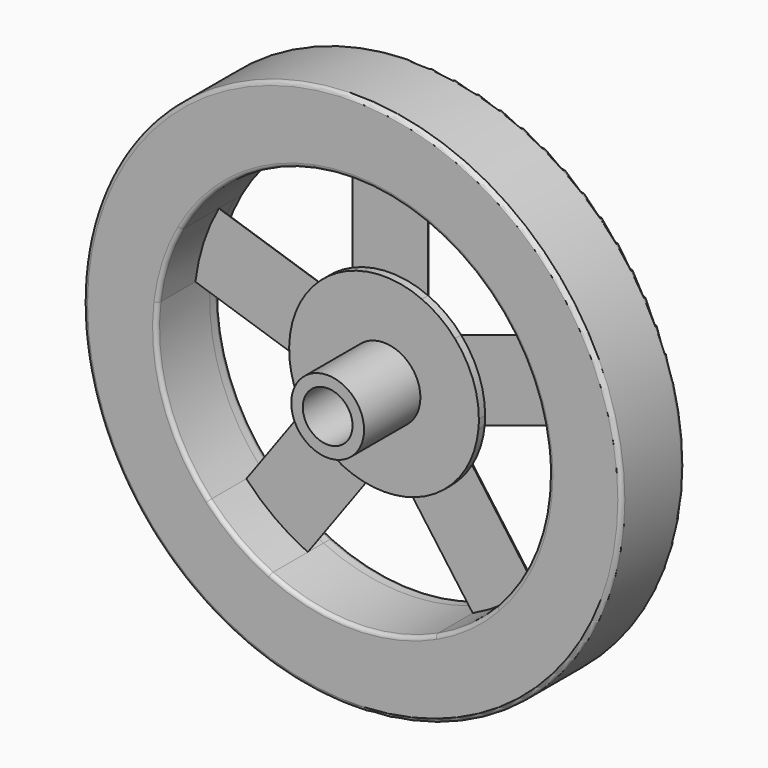
from build123d import *

# Parameters (mm, degrees)
F0_R          = 2.3622
F1_DEPTH      = 1.27
F2_T4_DEPTH   = 21.4195320699
F2_T9_DEPTH   = 21.4195320699
F2_T14_DEPTH  = 21.4195320699
F2_T19_DEPTH  = 21.4195320699
F2_T24_DEPTH  = 21.4195320699
F2_T29_DEPTH  = 21.4195320699
F2_T34_DEPTH  = 21.4195320699
F2_T39_DEPTH  = 21.4195320699
F2_T44_DEPTH  = 21.4195320699
F2_T49_DEPTH  = 21.4195320699
F2_T55_DEPTH  = 21.4195320699
F2_S57_R      = 2.3622
F2_T58_DEPTH  = 13
F2_T61_DEPTH  = 21.4195320699
F2_S63_R      = 2.3622
F2_T64_DEPTH  = 13
F2_T70_DEPTH  = 21.4195320699
F2_S72_R      = 2.3622
F2_T73_DEPTH  = 13
F2_T76_DEPTH  = 21.4195320699
F2_S78_R      = 2.3622
F2_T79_DEPTH  = 13
F2_T85_DEPTH  = 21.4195320699
F2_S87_R      = 2.3622
F2_T88_DEPTH  = 12
F2_T91_DEPTH  = 21.4195320699
F2_S93_R      = 2.3622
F2_T94_DEPTH  = 13
F2_T100_DEPTH = 21.4195320699
F2_S102_R     = 2.3622
F2_T103_DEPTH = 13
F2_T106_DEPTH = 21.4195320699
F2_S108_R     = 2.3622
F2_T109_DEPTH = 12
F2_T115_DEPTH = 21.4195320699
F2_S117_R     = 2.3622
F2_T118_DEPTH = 13
F2_T121_DEPTH = 21.4195320699
F2_S123_R     = 2.3622
F2_T124_DEPTH = 13
F0_R_2        = 17.4625
F3_DEPTH      = 4.318
F4_DEPTH      = 0.381
F5_DEPTH      = 0.762
F7_R          = 2.3622
F8_DEPTH      = 0.508
F7_R_2        = 1.6129
F9_DEPTH      = 5.08
F10_R         = 0.254


# Not quite as in the source:
# - a fillet or chamfer that OpenCascade refuses, or shapes differently, is made with other operations: its cross-section is extruded or revolved along the edge and cut away or added


with BuildPart() as f1:
    # F0 (on Front) → F1 (new body)
    with BuildSketch(Plane.XZ):
        with BuildLine():
            ThreePointArc((6.1303316445, -0.5987271324), (6.1522035895, -0.2997186064), (6.1595, 0))
            ThreePointArc((6.1595, 0), (5.7584751705, 2.1861847956), (4.607619503, 4.0876989573))
            Line((4.607619503, 4.0876989573), (2.4638, 3.3911297757))
            Line((2.4638, 3.3911297757), (2.4638, 5.6452749986))
            ThreePointArc((2.4638, 5.6452749986), (0, 6.1595), (-2.4638, 5.6452749986))
            Line((-2.4638, 5.6452749986), (-2.4638, 3.3911297757))
            Line((-2.4638, 3.3911297757), (-4.607619503, 4.0876989573))
            ThreePointArc((-4.607619503, 4.0876989573), (-5.8580326121, 1.9033901769), (-6.1303316445, -0.5987271324))
            Line((-6.1303316445, -0.5987271324), (-3.9865121415, -1.295296314))
            Line((-3.9865121415, -1.295296314), (-5.3114654601, -3.1189381072))
            ThreePointArc((-5.3114654601, -3.1189381072), (-3.6204632615, -4.9831401769), (-1.3249533186, -6.0153087164))
            Line((-1.3249533186, -6.0153087164), (0, -4.1916669232))
            Line((0, -4.1916669232), (1.3249533186, -6.0153087164))
            ThreePointArc((1.3249533186, -6.0153087164), (3.6204632615, -4.9831401769), (5.3114654601, -3.1189381072))
            Line((5.3114654601, -3.1189381072), (3.9865121415, -1.295296314))
            Line((3.9865121415, -1.295296314), (6.1303316445, -0.5987271324))
        make_face()
        Circle(F0_R, mode=Mode.SUBTRACT)
        with BuildLine():
            ThreePointArc((-2.4638, 5.6452749986), (0, 6.1595), (2.4638, 5.6452749986))
            Line((2.4638, 5.6452749986), (2.4638, 12.4975550077))
            ThreePointArc((2.4638, 12.4975550077), (0, 12.7381), (-2.4638, 12.4975550077))
            Line((-2.4638, 12.4975550077), (-2.4638, 5.6452749986))
        make_face()
        with BuildLine():
            Line((9.339134594, -8.6625490848), (5.3114654601, -3.1189381072))
            ThreePointArc((5.3114654601, -3.1189381072), (3.6204632615, -4.9831401769), (1.3249533186, -6.0153087164))
            Line((1.3249533186, -6.0153087164), (5.3526224525, -11.5589196939))
            ThreePointArc((5.3526224525, -11.5589196939), (7.4872673222, -10.305339376), (9.339134594, -8.6625490848))
        make_face()
        with BuildLine():
            Line((-5.3526224525, -11.5589196939), (-1.3249533186, -6.0153087164))
            ThreePointArc((-1.3249533186, -6.0153087164), (-3.6204632615, -4.9831401769), (-5.3114654601, -3.1189381072))
            Line((-5.3114654601, -3.1189381072), (-9.339134594, -8.6625490848))
            ThreePointArc((-9.339134594, -8.6625490848), (-7.4872673222, -10.305339376), (-5.3526224525, -11.5589196939))
        make_face()
        with BuildLine():
            ThreePointArc((-6.1303316445, -0.5987271324), (-5.8580326121, 1.9033901769), (-4.607619503, 4.0876989573))
            Line((-4.607619503, 4.0876989573), (-11.1245250571, 6.2051699304))
            ThreePointArc((-11.1245250571, 6.2051699304), (-12.1146530102, 3.936289376), (-12.6472371986, 1.5187438407))
            Line((-12.6472371986, 1.5187438407), (-6.1303316445, -0.5987271324))
        make_face()
        with BuildLine():
            ThreePointArc((4.607619503, 4.0876989573), (5.7584751705, 2.1861847956), (6.1595, 0))
            ThreePointArc((6.1595, 0), (6.1522035895, -0.2997186064), (6.1303316445, -0.5987271324))
            Line((6.1303316445, -0.5987271324), (12.6472371986, 1.5187438407))
            ThreePointArc((12.6472371986, 1.5187438407), (12.1146530102, 3.936289376), (11.1245250571, 6.2051699304))
            Line((11.1245250571, 6.2051699304), (4.607619503, 4.0876989573))
        make_face()
    extrude(amount=F1_DEPTH)

    # F2: fillet of radius 3.0226 on 10 edges, made by hand


with BuildPart() as f2_tool2:
    # F2_s3 → F2_t4 (new body)
    with BuildSketch(Plane(origin=(-10.9646098278, 0, -15.091490732), x_dir=(0, 1, 0), z_dir=(0.5877852523, 0, 0.8090169944))):
        with BuildLine():
            ThreePointArc((-1.27, -2.4638), (-0.3361972454, -1.386585071), (0, -0.0011786324))
            Line((0, -0.0011786324), (0, -2.4638))
            Line((0, -2.4638), (-1.27, -2.4638))
        make_face()
    extrude(amount=F2_T4_DEPTH)

    split(bisect_by=Plane(origin=(-1.9932560707, 0, -1.4481853046), x_dir=(0, 1, 0), z_dir=(-0.8090169944, 0, -0.5877852523)), keep=Keep.TOP)


with BuildPart() as f1_1:
    add(f1.part)

    # F2_t1: cut F2_tool2
    add(f2_tool2.part, mode=Mode.SUBTRACT)


with BuildPart() as f2_tool7:
    # F2_s8 → F2_t9 (new body)
    with BuildSketch(Plane(origin=(1.6254752339, 0, 2.237274724), x_dir=(0, 1, 0), z_dir=(-0.5877852523, 0, -0.8090169944))):
        with BuildLine():
            ThreePointArc((-1.27, -2.4638), (-0.3361972454, -1.386585071), (0, -0.0011786324))
            Line((0, -0.0011786324), (0, -2.4638))
            Line((0, -2.4638), (-1.27, -2.4638))
        make_face()
    extrude(amount=F2_T9_DEPTH)

    split(bisect_by=Plane(origin=(-0.7613560707, 0, -2.3432130448), x_dir=(0, 1, 0), z_dir=(-0.3090169944, 0, -0.9510565163)), keep=Keep.TOP)


with BuildPart() as f1_2:
    add(f1_1.part)

    # F2_t6: cut F2_tool7
    add(f2_tool7.part, mode=Mode.SUBTRACT)


with BuildPart() as f2_tool12:
    # F2_s13 → F2_t14 (new body)
    with BuildSketch(Plane(origin=(-17.7411113748, 0, 5.7644365187), x_dir=(0, 1, 0), z_dir=(0.9510565163, 0, -0.3090169944))):
        with BuildLine():
            ThreePointArc((-1.27, -2.4638), (-0.3361972454, -1.386585071), (0, -0.0011786324))
            Line((0, -0.0011786324), (0, -2.4638))
            Line((0, -2.4638), (-1.27, -2.4638))
        make_face()
    extrude(amount=F2_T14_DEPTH)

    split(bisect_by=Plane(origin=(-1.9932560707, 0, 1.4481853046), x_dir=(0, 1, 0), z_dir=(-0.8090169944, 0, 0.5877852523)), keep=Keep.TOP)


with BuildPart() as f1_3:
    add(f1_2.part)

    # F2_t11: cut F2_tool12
    add(f2_tool12.part, mode=Mode.SUBTRACT)


with BuildPart() as f2_tool17:
    # F2_s18 → F2_t19 (new body)
    with BuildSketch(Plane(origin=(2.6300741762, 0, -0.8545629024), x_dir=(0, 1, 0), z_dir=(-0.9510565163, 0, 0.3090169944))):
        with BuildLine():
            ThreePointArc((-1.27, -2.4638), (-0.3361972454, -1.386585071), (0, -0.0011786324))
            Line((0, -0.0011786324), (0, -2.4638))
            Line((0, -2.4638), (-1.27, -2.4638))
        make_face()
    extrude(amount=F2_T19_DEPTH)

    split(bisect_by=Plane.YZ.offset(-2.4638), keep=Keep.BOTTOM)


with BuildPart() as f1_4:
    add(f1_3.part)

    # F2_t16: cut F2_tool17
    add(f2_tool17.part, mode=Mode.SUBTRACT)


with BuildPart() as f2_tool22:
    # F2_s23 → F2_t24 (new body)
    with BuildSketch(Plane.XY.offset(-2.7654236433)):
        with BuildLine():
            ThreePointArc((2.4638, -1.27), (1.386585071, -0.3361972454), (0.0011786324, 0))
            Line((0.0011786324, 0), (2.4638, 0))
            Line((2.4638, 0), (2.4638, -1.27))
        make_face()
    extrude(amount=F2_T24_DEPTH)

    split(bisect_by=Plane(origin=(-0.7613560707, 0, 2.3432130448), x_dir=(0, 1, 0), z_dir=(-0.3090169944, 0, 0.9510565163)), keep=Keep.TOP)


with BuildPart() as f1_5:
    add(f1_4.part)

    # F2_t21: cut F2_tool22
    add(f2_tool22.part, mode=Mode.SUBTRACT)


with BuildPart() as f2_tool27:
    # F2_s28 → F2_t29 (new body)
    with BuildSketch(Plane.XY.offset(18.6541084266)):
        with BuildLine():
            ThreePointArc((-2.4638, -1.27), (-1.386585071, -0.3361972454), (-0.0011786324, 0))
            Line((-0.0011786324, 0), (-2.4638, 0))
            Line((-2.4638, 0), (-2.4638, -1.27))
        make_face()
    extrude(amount=-F2_T29_DEPTH)

    split(bisect_by=Plane(origin=(0.7613560707, 0, 2.3432130448), x_dir=(0, 1, 0), z_dir=(0.3090169944, 0, 0.9510565163)), keep=Keep.TOP)


with BuildPart() as f1_6:
    add(f1_5.part)

    # F2_t26: cut F2_tool27
    add(f2_tool27.part, mode=Mode.SUBTRACT)


with BuildPart() as f2_tool32:
    # F2_s33 → F2_t34 (new body)
    with BuildSketch(Plane(origin=(-2.6300741762, 0, -0.8545629024), x_dir=(0, 1, 0), z_dir=(0.9510565163, 0, 0.3090169944))):
        with BuildLine():
            ThreePointArc((-1.27, -2.4638), (-0.3361972454, -1.386585071), (0, -0.0011786324))
            Line((0, -0.0011786324), (0, -2.4638))
            Line((0, -2.4638), (-1.27, -2.4638))
        make_face()
    extrude(amount=F2_T34_DEPTH)

    split(bisect_by=Plane(origin=(1.9932560707, 0, 1.4481853046), x_dir=(0, 1, 0), z_dir=(0.8090169944, 0, 0.5877852523)), keep=Keep.TOP)


with BuildPart() as f1_7:
    add(f1_6.part)

    # F2_t31: cut F2_tool32
    add(f2_tool32.part, mode=Mode.SUBTRACT)


with BuildPart() as f2_tool37:
    # F2_s38 → F2_t39 (new body)
    with BuildSketch(Plane(origin=(17.7411113748, 0, 5.7644365187), x_dir=(0, 1, 0), z_dir=(-0.9510565163, 0, -0.3090169944))):
        with BuildLine():
            ThreePointArc((-1.27, -2.4638), (-0.3361972454, -1.386585071), (0, -0.0011786324))
            Line((0, -0.0011786324), (0, -2.4638))
            Line((0, -2.4638), (-1.27, -2.4638))
        make_face()
    extrude(amount=F2_T39_DEPTH)

    split(bisect_by=Plane.YZ.offset(2.4638), keep=Keep.TOP)


with BuildPart() as f1_8:
    add(f1_7.part)

    # F2_t36: cut F2_tool37
    add(f2_tool37.part, mode=Mode.SUBTRACT)


with BuildPart() as f2_tool42:
    # F2_s43 → F2_t44 (new body)
    with BuildSketch(Plane(origin=(10.9646098278, 0, -15.091490732), x_dir=(0, 1, 0), z_dir=(-0.5877852523, 0, 0.8090169944))):
        with BuildLine():
            ThreePointArc((-1.27, -2.4638), (-0.3361972454, -1.386585071), (0, -0.0011786324))
            Line((0, -0.0011786324), (0, -2.4638))
            Line((0, -2.4638), (-1.27, -2.4638))
        make_face()
    extrude(amount=F2_T44_DEPTH)

    split(bisect_by=Plane(origin=(0.7613560707, 0, -2.3432130448), x_dir=(0, 1, 0), z_dir=(0.3090169944, 0, -0.9510565163)), keep=Keep.TOP)


with BuildPart() as f1_9:
    add(f1_8.part)

    # F2_t41: cut F2_tool42
    add(f2_tool42.part, mode=Mode.SUBTRACT)


with BuildPart() as f2_tool47:
    # F2_s48 → F2_t49 (new body)
    with BuildSketch(Plane(origin=(-1.6254752339, 0, 2.237274724), x_dir=(0, 1, 0), z_dir=(0.5877852523, 0, -0.8090169944))):
        with BuildLine():
            ThreePointArc((-1.27, -2.4638), (-0.3361972454, -1.386585071), (0, -0.0011786324))
            Line((0, -0.0011786324), (0, -2.4638))
            Line((0, -2.4638), (-1.27, -2.4638))
        make_face()
    extrude(amount=F2_T49_DEPTH)

    split(bisect_by=Plane(origin=(1.9932560707, 0, -1.4481853046), x_dir=(0, 1, 0), z_dir=(0.8090169944, 0, -0.5877852523)), keep=Keep.TOP)


with BuildPart() as f1_10:
    add(f1_9.part)

    # F2_t46: cut F2_tool47
    add(f2_tool47.part, mode=Mode.SUBTRACT)


with BuildPart() as f2_tool53:
    # F2_s54 → F2_t55 (new body)
    with BuildSketch(Plane(origin=(-10.9646098278, 0, -15.091490732), x_dir=(0, 1, 0), z_dir=(0.5877852523, 0, 0.8090169944))):
        with BuildLine():
            ThreePointArc((-1.27, -2.4638), (-0.3361972454, -1.386585071), (0, -0.0011786324))
            Line((0, -0.0011786324), (0, -2.4638))
            Line((0, -2.4638), (-1.27, -2.4638))
        make_face()
    extrude(amount=F2_T55_DEPTH)

    split(bisect_by=Plane(origin=(-1.9932560707, 0, -1.4481853046), x_dir=(0, 1, 0), z_dir=(0.8090169944, 0, 0.5877852523)), keep=Keep.TOP)

    # F2_s57 → F2_t58 (cut, symmetric)
    with BuildSketch(Plane.XZ.offset(0.6)):
        Circle(F2_S57_R)
    extrude(amount=F2_T58_DEPTH, both=True, mode=Mode.SUBTRACT)


with BuildPart() as f2_tool59:
    # F2_s60 → F2_t61 (new body)
    with BuildSketch(Plane(origin=(-1.6254752339, 0, 2.237274724), x_dir=(0, 1, 0), z_dir=(0.5877852523, 0, -0.8090169944))):
        with BuildLine():
            ThreePointArc((-1.27, -2.4638), (-0.3361972454, -1.386585071), (0, -0.0011786324))
            Line((0, -0.0011786324), (0, -2.4638))
            Line((0, -2.4638), (-1.27, -2.4638))
        make_face()
    extrude(amount=F2_T61_DEPTH)

    split(bisect_by=Plane(origin=(1.9932560707, 0, -1.4481853046), x_dir=(0, 1, 0), z_dir=(-0.8090169944, 0, 0.5877852523)), keep=Keep.TOP)

    # F2_s63 → F2_t64 (cut, symmetric)
    with BuildSketch(Plane.XZ.offset(0.6)):
        Circle(F2_S63_R)
    extrude(amount=F2_T64_DEPTH, both=True, mode=Mode.SUBTRACT)


with BuildPart() as f2_tool53_1:
    add(f2_tool53.part)

    # F2_t65: intersect F2_tool59
    add(f2_tool59.part, mode=Mode.INTERSECT)


with BuildPart() as f1_11:
    add(f1_10.part)

    # F2_t51: cut F2_tool53
    add(f2_tool53_1.part, mode=Mode.SUBTRACT)


with BuildPart() as f2_tool68:
    # F2_s69 → F2_t70 (new body)
    with BuildSketch(Plane(origin=(-17.7411113748, 0, 5.7644365187), x_dir=(0, 1, 0), z_dir=(0.9510565163, 0, -0.3090169944))):
        with BuildLine():
            ThreePointArc((-1.27, -2.4638), (-0.3361972454, -1.386585071), (0, -0.0011786324))
            Line((0, -0.0011786324), (0, -2.4638))
            Line((0, -2.4638), (-1.27, -2.4638))
        make_face()
    extrude(amount=F2_T70_DEPTH)

    split(bisect_by=Plane(origin=(-1.9932560707, 0, 1.4481853046), x_dir=(0, 1, 0), z_dir=(0.8090169944, 0, -0.5877852523)), keep=Keep.TOP)

    # F2_s72 → F2_t73 (cut, symmetric)
    with BuildSketch(Plane.XZ.offset(0.6)):
        Circle(F2_S72_R)
    extrude(amount=F2_T73_DEPTH, both=True, mode=Mode.SUBTRACT)


with BuildPart() as f2_tool74:
    # F2_s75 → F2_t76 (new body)
    with BuildSketch(Plane(origin=(1.6254752339, 0, 2.237274724), x_dir=(0, 1, 0), z_dir=(-0.5877852523, 0, -0.8090169944))):
        with BuildLine():
            ThreePointArc((-1.27, -2.4638), (-0.3361972454, -1.386585071), (0, -0.0011786324))
            Line((0, -0.0011786324), (0, -2.4638))
            Line((0, -2.4638), (-1.27, -2.4638))
        make_face()
    extrude(amount=F2_T76_DEPTH)

    split(bisect_by=Plane(origin=(-0.7613560707, 0, -2.3432130448), x_dir=(0, 1, 0), z_dir=(0.3090169944, 0, 0.9510565163)), keep=Keep.TOP)

    # F2_s78 → F2_t79 (cut, symmetric)
    with BuildSketch(Plane.XZ.offset(0.6)):
        Circle(F2_S78_R)
    extrude(amount=F2_T79_DEPTH, both=True, mode=Mode.SUBTRACT)


with BuildPart() as f2_tool68_1:
    add(f2_tool68.part)

    # F2_t80: intersect F2_tool74
    add(f2_tool74.part, mode=Mode.INTERSECT)


with BuildPart() as f1_12:
    add(f1_11.part)

    # F2_t66: cut F2_tool68
    add(f2_tool68_1.part, mode=Mode.SUBTRACT)


with BuildPart() as f2_tool83:
    # F2_s84 → F2_t85 (new body)
    with BuildSketch(Plane.XY.offset(18.6541084266)):
        with BuildLine():
            ThreePointArc((-2.4638, -1.27), (-1.386585071, -0.3361972454), (-0.0011786324, 0))
            Line((-0.0011786324, 0), (-2.4638, 0))
            Line((-2.4638, 0), (-2.4638, -1.27))
        make_face()
    extrude(amount=-F2_T85_DEPTH)

    split(bisect_by=Plane(origin=(0.7613560707, 0, 2.3432130448), x_dir=(0, 1, 0), z_dir=(-0.3090169944, 0, -0.9510565163)), keep=Keep.TOP)

    # F2_s87 → F2_t88 (cut, symmetric)
    with BuildSketch(Plane.XZ.offset(0.6)):
        Circle(F2_S87_R)
    extrude(amount=F2_T88_DEPTH, both=True, mode=Mode.SUBTRACT)


with BuildPart() as f2_tool89:
    # F2_s90 → F2_t91 (new body)
    with BuildSketch(Plane(origin=(2.6300741762, 0, -0.8545629024), x_dir=(0, 1, 0), z_dir=(-0.9510565163, 0, 0.3090169944))):
        with BuildLine():
            ThreePointArc((-1.27, -2.4638), (-0.3361972454, -1.386585071), (0, -0.0011786324))
            Line((0, -0.0011786324), (0, -2.4638))
            Line((0, -2.4638), (-1.27, -2.4638))
        make_face()
    extrude(amount=F2_T91_DEPTH)

    split(bisect_by=Plane.YZ.offset(-2.4638), keep=Keep.TOP)

    # F2_s93 → F2_t94 (cut, symmetric)
    with BuildSketch(Plane.XZ.offset(0.6)):
        Circle(F2_S93_R)
    extrude(amount=F2_T94_DEPTH, both=True, mode=Mode.SUBTRACT)


with BuildPart() as f2_tool83_1:
    add(f2_tool83.part)

    # F2_t95: intersect F2_tool89
    add(f2_tool89.part, mode=Mode.INTERSECT)


with BuildPart() as f1_13:
    add(f1_12.part)

    # F2_t81: cut F2_tool83
    add(f2_tool83_1.part, mode=Mode.SUBTRACT)


with BuildPart() as f2_tool98:
    # F2_s99 → F2_t100 (new body)
    with BuildSketch(Plane(origin=(17.7411113748, 0, 5.7644365187), x_dir=(0, 1, 0), z_dir=(-0.9510565163, 0, -0.3090169944))):
        with BuildLine():
            ThreePointArc((-1.27, -2.4638), (-0.3361972454, -1.386585071), (0, -0.0011786324))
            Line((0, -0.0011786324), (0, -2.4638))
            Line((0, -2.4638), (-1.27, -2.4638))
        make_face()
    extrude(amount=F2_T100_DEPTH)

    split(bisect_by=Plane.YZ.offset(2.4638), keep=Keep.BOTTOM)

    # F2_s102 → F2_t103 (cut, symmetric)
    with BuildSketch(Plane.XZ.offset(0.6)):
        Circle(F2_S102_R)
    extrude(amount=F2_T103_DEPTH, both=True, mode=Mode.SUBTRACT)


with BuildPart() as f2_tool104:
    # F2_s105 → F2_t106 (new body)
    with BuildSketch(Plane.XY.offset(-2.7654236433)):
        with BuildLine():
            ThreePointArc((2.4638, -1.27), (1.386585071, -0.3361972454), (0.0011786324, 0))
            Line((0.0011786324, 0), (2.4638, 0))
            Line((2.4638, 0), (2.4638, -1.27))
        make_face()
    extrude(amount=F2_T106_DEPTH)

    split(bisect_by=Plane(origin=(-0.7613560707, 0, 2.3432130448), x_dir=(0, 1, 0), z_dir=(0.3090169944, 0, -0.9510565163)), keep=Keep.TOP)

    # F2_s108 → F2_t109 (cut, symmetric)
    with BuildSketch(Plane.XZ.offset(0.6)):
        Circle(F2_S108_R)
    extrude(amount=F2_T109_DEPTH, both=True, mode=Mode.SUBTRACT)


with BuildPart() as f2_tool98_1:
    add(f2_tool98.part)

    # F2_t110: intersect F2_tool104
    add(f2_tool104.part, mode=Mode.INTERSECT)


with BuildPart() as f1_14:
    add(f1_13.part)

    # F2_t96: cut F2_tool98
    add(f2_tool98_1.part, mode=Mode.SUBTRACT)


with BuildPart() as f2_tool113:
    # F2_s114 → F2_t115 (new body)
    with BuildSketch(Plane(origin=(-2.6300741762, 0, -0.8545629024), x_dir=(0, 1, 0), z_dir=(0.9510565163, 0, 0.3090169944))):
        with BuildLine():
            ThreePointArc((-1.27, -2.4638), (-0.3361972454, -1.386585071), (0, -0.0011786324))
            Line((0, -0.0011786324), (0, -2.4638))
            Line((0, -2.4638), (-1.27, -2.4638))
        make_face()
    extrude(amount=F2_T115_DEPTH)

    split(bisect_by=Plane(origin=(1.9932560707, 0, 1.4481853046), x_dir=(0, 1, 0), z_dir=(-0.8090169944, 0, -0.5877852523)), keep=Keep.TOP)

    # F2_s117 → F2_t118 (cut, symmetric)
    with BuildSketch(Plane.XZ.offset(0.6)):
        Circle(F2_S117_R)
    extrude(amount=F2_T118_DEPTH, both=True, mode=Mode.SUBTRACT)


with BuildPart() as f2_tool119:
    # F2_s120 → F2_t121 (new body)
    with BuildSketch(Plane(origin=(10.9646098278, 0, -15.091490732), x_dir=(0, 1, 0), z_dir=(-0.5877852523, 0, 0.8090169944))):
        with BuildLine():
            ThreePointArc((-1.27, -2.4638), (-0.3361972454, -1.386585071), (0, -0.0011786324))
            Line((0, -0.0011786324), (0, -2.4638))
            Line((0, -2.4638), (-1.27, -2.4638))
        make_face()
    extrude(amount=F2_T121_DEPTH)

    split(bisect_by=Plane(origin=(0.7613560707, 0, -2.3432130448), x_dir=(0, 1, 0), z_dir=(-0.3090169944, 0, 0.9510565163)), keep=Keep.TOP)

    # F2_s123 → F2_t124 (cut, symmetric)
    with BuildSketch(Plane.XZ.offset(0.6)):
        Circle(F2_S123_R)
    extrude(amount=F2_T124_DEPTH, both=True, mode=Mode.SUBTRACT)


with BuildPart() as f2_tool113_1:
    add(f2_tool113.part)

    # F2_t125: intersect F2_tool119
    add(f2_tool119.part, mode=Mode.INTERSECT)


with BuildPart() as f1_15:
    add(f1_14.part)

    # F2_t111: cut F2_tool113
    add(f2_tool113_1.part, mode=Mode.SUBTRACT)

    # F0 (on Front) → F3 (join)
    with BuildSketch(Plane.XZ):
        Circle(F0_R_2)
        with BuildLine():
            ThreePointArc((2.4638, 12.4975550077), (7.4872673222, 10.305339376), (11.1245250571, 6.2051699304))
            ThreePointArc((11.1245250571, 6.2051699304), (12.1146530102, 3.936289376), (12.6472371986, 1.5187438407))
            ThreePointArc((12.6472371986, 1.5187438407), (12.7153640091, 0.7607297323), (12.7381, 0))
            ThreePointArc((12.7381, 0), (11.8579513825, -4.6527605375), (9.339134594, -8.6625490848))
            ThreePointArc((9.339134594, -8.6625490848), (7.4872673222, -10.305339376), (5.3526224525, -11.5589196939))
            ThreePointArc((5.3526224525, -11.5589196939), (0, -12.7381), (-5.3526224525, -11.5589196939))
            ThreePointArc((-5.3526224525, -11.5589196939), (-7.4872673222, -10.305339376), (-9.339134594, -8.6625490848))
            ThreePointArc((-9.339134594, -8.6625490848), (-12.1146530102, -3.936289376), (-12.6472371986, 1.5187438407))
            ThreePointArc((-12.6472371986, 1.5187438407), (-12.1146530102, 3.936289376), (-11.1245250571, 6.2051699304))
            ThreePointArc((-11.1245250571, 6.2051699304), (-7.4872673222, 10.305339376), (-2.4638, 12.4975550077))
            ThreePointArc((-2.4638, 12.4975550077), (0, 12.7381), (2.4638, 12.4975550077))
        make_face(mode=Mode.SUBTRACT)
    extrude(amount=F3_DEPTH)

    # F0 (on Front) → F4 (join, symmetric)
    with BuildSketch(Plane.XZ):
        Circle(F0_R)
    extrude(amount=F4_DEPTH, both=True)

    # F0 (on Front) → F5 (join)
    with BuildSketch(Plane.XZ):
        Circle(F0_R_2)
        with BuildLine():
            ThreePointArc((2.4638, 12.4975550077), (7.4872673222, 10.305339376), (11.1245250571, 6.2051699304))
            ThreePointArc((11.1245250571, 6.2051699304), (12.1146530102, 3.936289376), (12.6472371986, 1.5187438407))
            ThreePointArc((12.6472371986, 1.5187438407), (12.7153640091, 0.7607297323), (12.7381, 0))
            ThreePointArc((12.7381, 0), (11.8579513825, -4.6527605375), (9.339134594, -8.6625490848))
            ThreePointArc((9.339134594, -8.6625490848), (7.4872673222, -10.305339376), (5.3526224525, -11.5589196939))
            ThreePointArc((5.3526224525, -11.5589196939), (0, -12.7381), (-5.3526224525, -11.5589196939))
            ThreePointArc((-5.3526224525, -11.5589196939), (-7.4872673222, -10.305339376), (-9.339134594, -8.6625490848))
            ThreePointArc((-9.339134594, -8.6625490848), (-12.1146530102, -3.936289376), (-12.6472371986, 1.5187438407))
            ThreePointArc((-12.6472371986, 1.5187438407), (-12.1146530102, 3.936289376), (-11.1245250571, 6.2051699304))
            ThreePointArc((-11.1245250571, 6.2051699304), (-7.4872673222, 10.305339376), (-2.4638, 12.4975550077))
            ThreePointArc((-2.4638, 12.4975550077), (0, 12.7381), (2.4638, 12.4975550077))
        make_face(mode=Mode.SUBTRACT)
    extrude(amount=-F5_DEPTH)

    # F6: fillet of radius 0.508 on 1 edges, made by hand

    # F6_s1 → F6_t2 (revolve, cut)
    with BuildSketch(Plane.XY):
        with BuildLine():
            ThreePointArc((2.3622, -0.127), (2.2134102448, 0.2322102448), (1.8542, 0.381))
            Line((1.8542, 0.381), (2.3622, 0.381))
            Line((2.3622, 0.381), (2.3622, -0.127))
        make_face()
    revolve(axis=Axis((0, 0.381, 0), (0, -1, 0)), mode=Mode.SUBTRACT)

    # F7 (on face) → F8 (join)
    with BuildSketch(Plane.XZ.offset(1.27)):
        with BuildLine():
            ThreePointArc((6.127971625, -0.5994939492), (6.149907888, -0.3001036489), (6.157225774, 0))
            ThreePointArc((6.157225774, 0), (5.756172844, 2.1858415821), (4.6052594835, 4.0869321405))
            Line((4.6052594835, 4.0869321405), (2.4638, 3.3911297757))
            Line((2.4638, 3.3911297757), (2.4638, 5.6427935273))
            ThreePointArc((2.4638, 5.6427935273), (0, 6.157225774), (-2.4638, 5.6427935273))
            Line((-2.4638, 5.6427935273), (-2.4638, 3.3911297757))
            Line((-2.4638, 3.3911297757), (-4.6052594835, 4.0869321405))
            ThreePointArc((-4.6052594835, 4.0869321405), (-5.8558696946, 1.9026874024), (-6.127971625, -0.5994939492))
            Line((-6.127971625, -0.5994939492), (-3.9865121415, -1.295296314))
            Line((-3.9865121415, -1.295296314), (-5.3100068878, -3.1169305547))
            ThreePointArc((-5.3100068878, -3.1169305547), (-3.619126505, -4.9813002893), (-1.3234947463, -6.0133011639))
            Line((-1.3234947463, -6.0133011639), (0, -4.1916669232))
            Line((0, -4.1916669232), (1.3234947463, -6.0133011639))
            ThreePointArc((1.3234947463, -6.0133011639), (3.619126505, -4.9813002893), (5.3100068878, -3.1169305547))
            Line((5.3100068878, -3.1169305547), (3.9865121415, -1.295296314))
            Line((3.9865121415, -1.295296314), (6.127971625, -0.5994939492))
        make_face()
        Circle(F7_R, mode=Mode.SUBTRACT)
        with BuildLine():
            Line((-2.4638, 3.3911297757), (-2.4638, 5.6427935273))
            ThreePointArc((-2.4638, 5.6427935273), (-3.619126505, 4.9813002893), (-4.6052594835, 4.0869321405))
            Line((-4.6052594835, 4.0869321405), (-2.4638, 3.3911297757))
        make_face()
        with BuildLine():
            Line((2.4638, 3.3911297757), (4.6052594835, 4.0869321405))
            ThreePointArc((4.6052594835, 4.0869321405), (3.619126505, 4.9813002893), (2.4638, 5.6427935273))
            Line((2.4638, 5.6427935273), (2.4638, 3.3911297757))
        make_face()
        with BuildLine():
            Line((-3.9865121415, -1.295296314), (-6.127971625, -0.5994939492))
            ThreePointArc((-6.127971625, -0.5994939492), (-5.8558696946, -1.9026874024), (-5.3100068878, -3.1169305547))
            Line((-5.3100068878, -3.1169305547), (-3.9865121415, -1.295296314))
        make_face()
        with BuildLine():
            ThreePointArc((-1.3234947463, -6.0133011639), (0, -6.157225774), (1.3234947463, -6.0133011639))
            Line((1.3234947463, -6.0133011639), (0, -4.1916669232))
            Line((0, -4.1916669232), (-1.3234947463, -6.0133011639))
        make_face()
        with BuildLine():
            ThreePointArc((5.3100068878, -3.1169305547), (5.8558696946, -1.9026874024), (6.127971625, -0.5994939492))
            Line((6.127971625, -0.5994939492), (3.9865121415, -1.295296314))
            Line((3.9865121415, -1.295296314), (5.3100068878, -3.1169305547))
        make_face()
    extrude(amount=F8_DEPTH)

    # F7 (on face) → F9 (join)
    with BuildSketch(Plane.XZ.offset(1.27)):
        Circle(F7_R)
        Circle(F7_R_2, mode=Mode.SUBTRACT)
    extrude(amount=F9_DEPTH)

    # F10
    f10_edges = [f1_15.edges().sort_by_distance(p)[0] for p in [
        (-17.4625, 0.762, 0),
        (-17.4625, -4.318, 0),
        (-9.339135, 0.762, 8.662549),
        (-9.339135, -4.318, 8.662549),
    ]]
    fillet(f10_edges, radius=F10_R)


solid = f1_15.part
